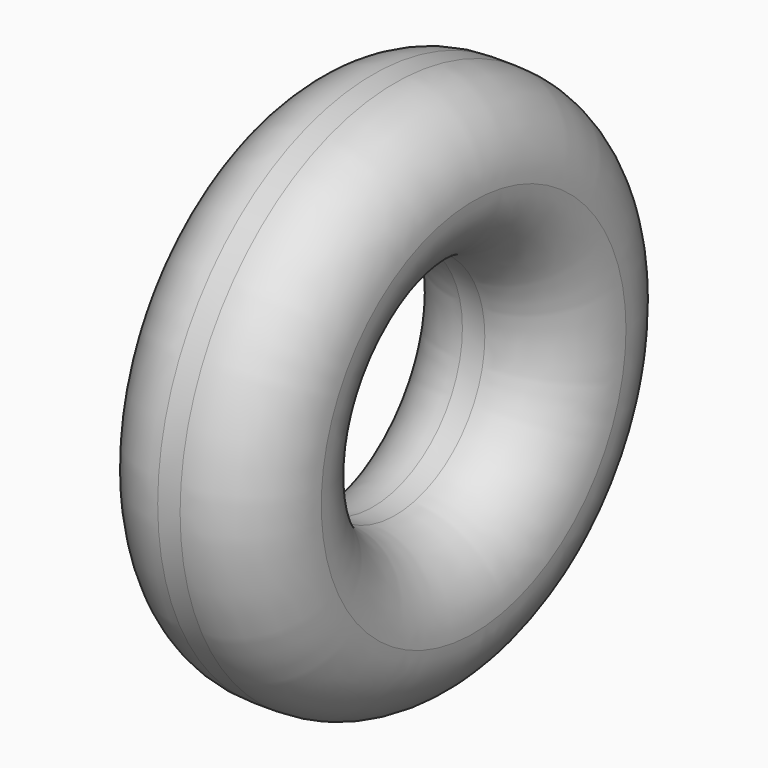
from build123d import *

# Parameters (mm, degrees)
F0_R     = 6
F0_R_2   = 2.5
F1_DEPTH = 4
F2_R     = 1.74999


# Not quite as in the source:
# - a fillet or chamfer is up to 0.001 mm smaller than in the source, because OpenCascade refuses the exact size


with BuildPart() as f1:
    # F0 (on Right) → F1 (new body)
    with BuildSketch(Plane.YZ):
        Circle(F0_R)
        Circle(F0_R_2, mode=Mode.SUBTRACT)
    extrude(amount=F1_DEPTH)

    # F2 (radius 1.75 in the source; OpenCascade refuses exactly that, so slightly less here)
    f2_edges = [f1.edges().sort_by_distance(p)[0] for p in [
        (4, -6, 0),
        (4, -2.5, 0),
        (0, -6, 0),
        (0, -2.5, 0),
    ]]
    fillet(f2_edges, radius=F2_R)


solid = f1.part
